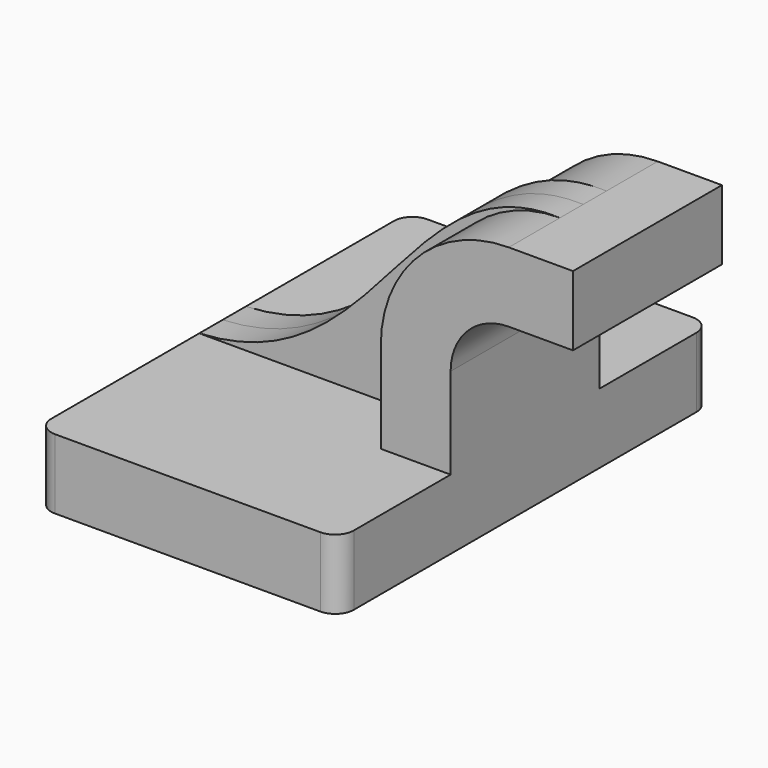
from build123d import *

# Parameters (mm, degrees)
F1_DEPTH = 63.5
F0_W     = 2.669878304
F0_H     = 19.05
F2_DEPTH = 25.4
F3_DEPTH = 7.9375
F5_R     = 5.08


# Not quite as in the source:
# - a feature of the source that left no trace in its solid (it failed there, or was rolled back) is left out


with BuildPart() as f1:
    # F0 (on Front) → F1 (new body, symmetric)
    with BuildSketch(Plane.XZ):
        Polygon((22.225, 9.525), (-41.275, 9.525), (-41.275, -9.525), (41.275, -9.525), (41.275, 9.525), align=None)
    extrude(amount=F1_DEPTH, both=True)

    # F0 (on Front) → F2 (join, symmetric)
    with BuildSketch(Plane.XZ):
        with BuildLine():
            Line((22.225, 34.3503219656), (22.225, 9.525))
            Line((22.225, 9.525), (41.275, 9.525))
            Line((41.275, 9.525), (41.275, 34.3503219656))
            ThreePointArc((41.275, 34.3503219656), (45.9246798487, 45.5756421169), (57.15, 50.2253219656))
            Line((57.15, 50.2253219656), (71.9948219351, 50.2253219656))
            Line((71.9948219351, 50.2253219656), (71.9948219351, 69.2753219656))
            Line((71.9948219351, 69.2753219656), (57.15, 69.2753219656))
            ThreePointArc((57.15, 69.2753219656), (32.4542956671, 59.0460262985), (22.225, 34.3503219656))
        make_face()
        with Locations((73.3297610871, 59.7503219656)):
            Rectangle(F0_W, F0_H)
    extrude(amount=F2_DEPTH, both=True)

    # F0 (on Front) → F3 (join, symmetric)
    with BuildSketch(Plane.XZ):
        with BuildLine():
            add(Edge.make_bspline(
                [(-41.275, 9.525), (8.1134410575, 11.8744410574), (14.8591641337, 70.7333981991), (57.15, 69.2753219656)],
                knots=[0, 0, 0, 0, 115.1415719885, 115.1415719885, 115.1415719885, 115.1415719885], degree=3))
            Line((-41.275, 9.525), (22.225, 9.525))
            Line((22.225, 9.525), (22.225, 34.3503219656))
            ThreePointArc((22.225, 34.3503219656), (32.4542956671, 59.0460262985), (57.15, 69.2753219656))
        make_face()
    extrude(amount=F3_DEPTH, both=True)

    # F5
    f5_edges = [f1.edges().sort_by_distance(p)[0] for p in [
        (-41.275, -63.5, 0),
        (-41.275, 63.5, 0),
        (41.275, -63.5, 0),
        (41.275, 63.5, 0),
    ]]
    fillet(f5_edges, radius=F5_R)


solid = f1.part
